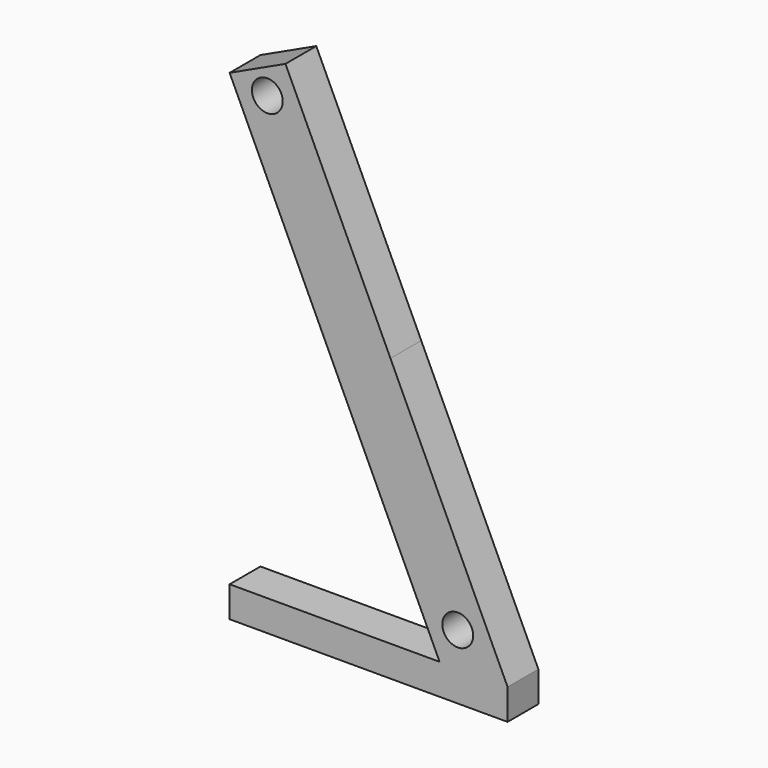
from build123d import *

# Parameters (mm, degrees)
F0_R     = 2
F1_DEPTH = 5


# Not quite as in the source:
# - a feature names something its author has since deleted; it is built from what else it names


with BuildPart() as f1:
    # F0 (on Front) → F1 (new body)
    with BuildSketch(Plane.XZ):
        Polygon((-8.8270233517, 0), (-36.085901234, 0), (-36.085901234, -4), (0, -4), (0, 0), (-15.2059999965, 32.6093722259), (-22.4564622928, 29.2284261319), align=None)
        with Locations((-6.4696469888, 4.4093964081)):
            Circle(F0_R, mode=Mode.SUBTRACT)
        Polygon((-36.085901234, 58.4568522639), (-22.4564622928, 29.2284261319), (-15.2059999965, 32.6093722259), (-28.8354389377, 61.8377983578), align=None)
        with Locations((-31.1928153006, 57.4284019497)):
            Circle(F0_R, mode=Mode.SUBTRACT)
    extrude(amount=F1_DEPTH)


solid = f1.part
